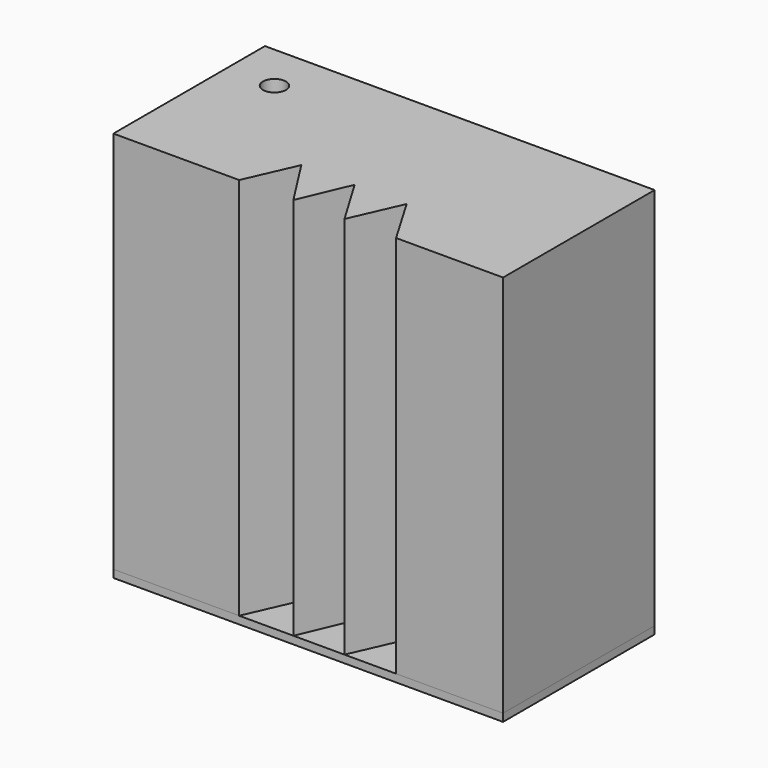
from build123d import *

# Parameters (mm, degrees)
F0_W     = 50.8
F0_H     = 24.7
F1_DEPTH = 1
F2_R     = 1.5
F3_DEPTH = 25
F4_R     = 1.5
F5_DEPTH = 25
F6_DEPTH = 25


# Not quite as in the source:
# - a feature of the source that left no trace in its solid (it failed there, or was rolled back) is left out


with BuildPart() as f1:
    # F0 (on Top) → F1 (new body)
    with BuildSketch(Plane.XY):
        Rectangle(F0_W, F0_H)
    extrude(amount=F1_DEPTH)

    # F2 (on face) → F3 (cut)
    with BuildSketch(Plane.XY.offset(1)):
        with Locations((-19.1877838224, 6.1313840561)):
            Circle(F2_R)
    extrude(amount=-F3_DEPTH, mode=Mode.SUBTRACT)


with BuildPart() as f5:
    # F4 (on face) → F5 (new body)
    with BuildSketch(Plane.XY.offset(1)):
        Polygon((-25.4, -12.35), (-9.0006701648, -12.35), (-6.1190491542, -5.8241537772), (-1.9378731959, -12.35), (0.8307432872, -5.8241537772), (4.7294073738, -12.35), (7.6110288501, -5.8241537772), (11.4531898871, -12.35), (25.4, -12.35), (25.4, 12.35), (-25.4, 12.35), align=None)
        with Locations((-19.1877838224, 6.1313840561)):
            Circle(F4_R, mode=Mode.SUBTRACT)
    extrude(amount=F5_DEPTH)

    # F6 (add): a face of the model
    f6_faces = [f5.faces().sort_by_distance(p)[0] for p in [
        (0.0562187638, 0.5383064409, 26),
    ]]
    extrude(f6_faces, amount=F6_DEPTH)


solid = Compound([f1.part, f5.part])
